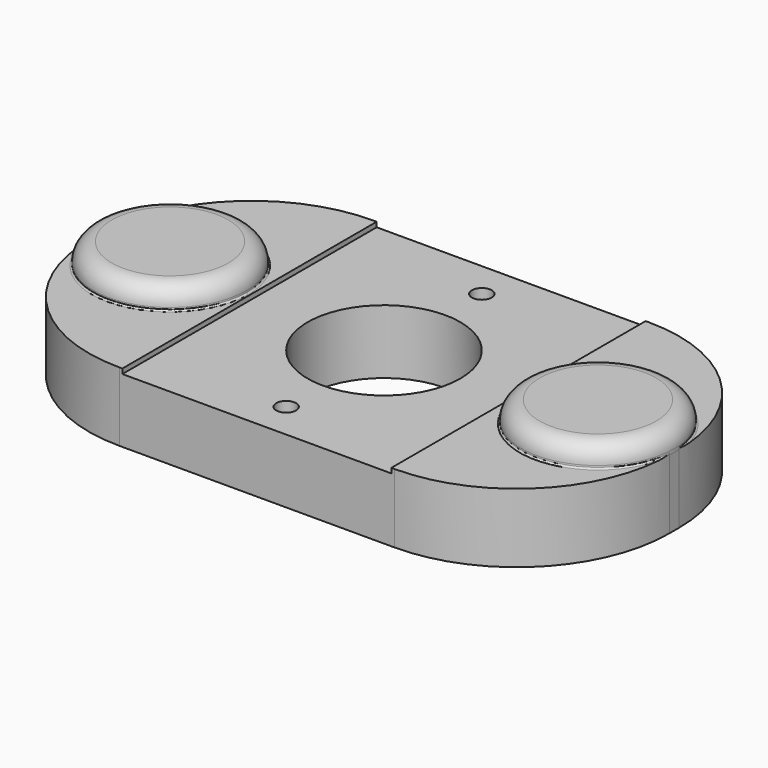
from build123d import *

# Parameters (mm, degrees)
F0_R          = 1.625
F1_DEPTH      = 11.3
F2_R          = 12.5
F3_DEPTH      = 11.301
F4_R          = 9.5
F5_DEPTH      = 10.5
F6_R          = 3.125
F7_DEPTH      = 5
F8_W          = 44
F8_H          = 52
F9_DEPTH      = 0.8
F10_R         = 12.539936204
F10_R_2       = 9.5
F11_DEPTH     = 1
F12_R         = 12.54
F13_DEPTH     = 2.5
F16_T4_ANGLE  = 178.2861059353
F16_S5_R      = 25
F16_T6_DEPTH  = 17
F16_T10_ANGLE = 178.2861059353
F16_S11_R     = 25
F16_T12_DEPTH = 17
F16_T16_ANGLE = 356.5984947452
F16_S17_R     = 25
F16_T18_DEPTH = 21
F16_T22_ANGLE = 356.5984947452
F16_S23_R     = 25
F16_T24_DEPTH = 21


# Not quite as in the source:
# - a fillet or chamfer that OpenCascade refuses, or shapes differently, is made with other operations: its cross-section is extruded or revolved along the edge and cut away or added
# - a feature of the source that left no trace in its solid (it failed there, or was rolled back) is left out


with BuildPart() as f1:
    # F0 (on Top) → F1 (new body)
    with BuildSketch(Plane.XY):
        with BuildLine():
            Line((-22.5, -26), (22.5, -26))
            ThreePointArc((22.5, -26), (40.1776695297, -18.6776695297), (47.5, -1))
            Line((47.5, -1), (47.5, 1))
            ThreePointArc((47.5, 1), (40.1776695297, 18.6776695297), (22.5, 26))
            Line((22.5, 26), (-22.5, 26))
            ThreePointArc((-22.5, 26), (-40.1776695297, 18.6776695297), (-47.5, 1))
            Line((-47.5, 1), (-47.5, -1))
            ThreePointArc((-47.5, -1), (-40.1776695297, -18.6776695297), (-22.5, -26))
        make_face()
        with Locations((0, -20)):
            Circle(F0_R, mode=Mode.SUBTRACT)
        with Locations((0, 20)):
            Circle(F0_R, mode=Mode.SUBTRACT)
    extrude(amount=F1_DEPTH)

    # F2 (on face) → F3 (cut, through all)
    with BuildSketch(Plane(origin=(0, 0, 0), x_dir=(1, 0, 0), z_dir=(0, 0, -1))):
        Circle(F2_R)
    extrude(amount=-F3_DEPTH, mode=Mode.SUBTRACT)

    # F4 (on face) → F5 (cut)
    with BuildSketch(Plane.XY.offset(11.3)):
        with Locations((-35, 0)):
            Circle(F4_R)
        with Locations((35, 0)):
            Circle(F4_R)
    extrude(amount=-F5_DEPTH, mode=Mode.SUBTRACT)

    # F6 (on face) → F7 (cut)
    with BuildSketch(Plane(origin=(0, 0, 0), x_dir=(1, 0, 0), z_dir=(0, 0, -1))):
        with Locations((0, 20)):
            Circle(F6_R)
        with Locations((0, -20)):
            Circle(F6_R)
    extrude(amount=-F7_DEPTH, mode=Mode.SUBTRACT)

    # F8 (on face) → F9 (cut)
    with BuildSketch(Plane.XY.offset(11.3)):
        Rectangle(F8_W, F8_H)
    extrude(amount=-F9_DEPTH, mode=Mode.SUBTRACT)

    # F10 (on face) → F11 (join)
    with BuildSketch(Plane.XY.offset(11.3)):
        with Locations((-35, 0)):
            Circle(F10_R)
        with Locations((-35, 0)):
            Circle(F10_R_2, mode=Mode.SUBTRACT)
        with Locations((35, 0)):
            Circle(F10_R)
        with Locations((35, 0)):
            Circle(F10_R_2, mode=Mode.SUBTRACT)
    extrude(amount=F11_DEPTH)

    # F12 (on face) → F13 (join)
    with BuildSketch(Plane.XY.offset(12.3)):
        with Locations((-35, 0)):
            Circle(F12_R)
        with Locations((35, 0)):
            Circle(F12_R)
    extrude(amount=F13_DEPTH)

    # F14: fillet of radius 3 on 1 edges, made by hand

    # F14_s1 → F14_t2 (revolve, cut)
    with BuildSketch(Plane.XZ):
        with BuildLine():
            ThreePointArc((-22.46, 11.8), (-23.3386796564, 13.9213203436), (-25.46, 14.8))
            Line((-25.46, 14.8), (-22.46, 14.8))
            Line((-22.46, 14.8), (-22.46, 11.8))
        make_face()
    revolve(axis=Axis((-35, 0, 14.8), (0, 0, 1)), mode=Mode.SUBTRACT)

    # F15: fillet of radius 3 on 1 edges, made by hand

    # F15_s1 → F15_t2 (revolve, cut)
    with BuildSketch(Plane.XZ):
        with BuildLine():
            ThreePointArc((47.54, 11.8), (46.6613203436, 13.9213203436), (44.54, 14.8))
            Line((44.54, 14.8), (47.54, 14.8))
            Line((47.54, 14.8), (47.54, 11.8))
        make_face()
    revolve(axis=Axis((35, 0, 14.8), (0, 0, 1)), mode=Mode.SUBTRACT)

    # F16: fillet of radius 0.25 on 3 edges, made by hand


with BuildPart() as f16_tool2:
    # F16_s3 → F16_t4 (revolve)
    with BuildSketch(Plane.XZ):
        with BuildLine():
            ThreePointArc((-22.460063796, 11.55), (-22.3868404913, 11.3732233047), (-22.210063796, 11.3))
            Line((-22.210063796, 11.3), (-22.460063796, 11.3))
            Line((-22.460063796, 11.3), (-22.460063796, 11.55))
        make_face()
    revolve(axis=Axis((-35, 0, 11.3), (0, 0, 1)), revolution_arc=F16_T4_ANGLE)

    # F16_s5 → F16_t6 (intersect, symmetric)
    with BuildSketch(Plane.XY.offset(11.5)):
        with Locations((-22.5, 1)):
            Circle(F16_S5_R)
    extrude(amount=F16_T6_DEPTH, both=True, mode=Mode.INTERSECT)


with BuildPart() as f1_1:
    add(f1.part)

    # F16_t1: union F16_tool2
    add(f16_tool2.part)


with BuildPart() as f16_tool8:
    # F16_s9 → F16_t10 (revolve)
    with BuildSketch(Plane(origin=(-0.0313084228, 1.046333877, 0), x_dir=(0, 0, 1), z_dir=(-0.0299086337, 0.9995526367, 0))):
        with BuildLine():
            ThreePointArc((11.55, -47.5242784902), (11.3732233047, -47.5975017949), (11.3, -47.7742784902))
            Line((11.3, -47.7742784902), (11.3, -47.5242784902))
            Line((11.3, -47.5242784902), (11.55, -47.5242784902))
        make_face()
    revolve(axis=Axis((-35, 0, 11.3), (0, 0, 1)), revolution_arc=F16_T10_ANGLE)

    # F16_s11 → F16_t12 (intersect, symmetric)
    with BuildSketch(Plane.XY.offset(11.5)):
        with Locations((-22.5, -1)):
            Circle(F16_S11_R)
    extrude(amount=F16_T12_DEPTH, both=True, mode=Mode.INTERSECT)


with BuildPart() as f1_2:
    add(f1_1.part)

    # F16_t7: union F16_tool8
    add(f16_tool8.part)


with BuildPart() as f16_tool14:
    # F16_s15 → F16_t16 (revolve)
    with BuildSketch(Plane(origin=(0.0308302837, -1.0383204819, 0), x_dir=(0, 0, 1), z_dir=(0.0296793741, -0.9995594703, 0))):
        with BuildLine():
            ThreePointArc((11.55, -47.524517666), (11.3732233047, -47.5977409707), (11.3, -47.774517666))
            Line((11.3, -47.774517666), (11.3, -47.524517666))
            Line((11.3, -47.524517666), (11.55, -47.524517666))
        make_face()
    revolve(axis=Axis((35, 0, 11.3), (0, 0, 1)), revolution_arc=F16_T16_ANGLE)

    # F16_s17 → F16_t18 (intersect, symmetric)
    with BuildSketch(Plane.XY.offset(11.5)):
        with Locations((22.5, 1)):
            Circle(F16_S17_R)
    extrude(amount=F16_T18_DEPTH, both=True, mode=Mode.INTERSECT)


with BuildPart() as f1_3:
    add(f1_2.part)

    # F16_t13: union F16_tool14
    add(f16_tool14.part)


with BuildPart() as f16_tool20:
    # F16_s21 → F16_t22 (revolve)
    with BuildSketch(Plane(origin=(0.0308302837, -1.0383204819, 0), x_dir=(0, 0, 1), z_dir=(0.0296793741, -0.9995594703, 0))):
        with BuildLine():
            ThreePointArc((11.55, -47.524517666), (11.3732233047, -47.5977409707), (11.3, -47.774517666))
            Line((11.3, -47.774517666), (11.3, -47.524517666))
            Line((11.3, -47.524517666), (11.55, -47.524517666))
        make_face()
    revolve(axis=Axis((35, 0, 11.3), (0, 0, 1)), revolution_arc=F16_T22_ANGLE)

    # F16_s23 → F16_t24 (intersect, symmetric)
    with BuildSketch(Plane.XY.offset(11.5)):
        with Locations((22.5, -1)):
            Circle(F16_S23_R)
    extrude(amount=F16_T24_DEPTH, both=True, mode=Mode.INTERSECT)


with BuildPart() as f1_4:
    add(f1_3.part)

    # F16_t19: union F16_tool20
    add(f16_tool20.part)


solid = f1_4.part
